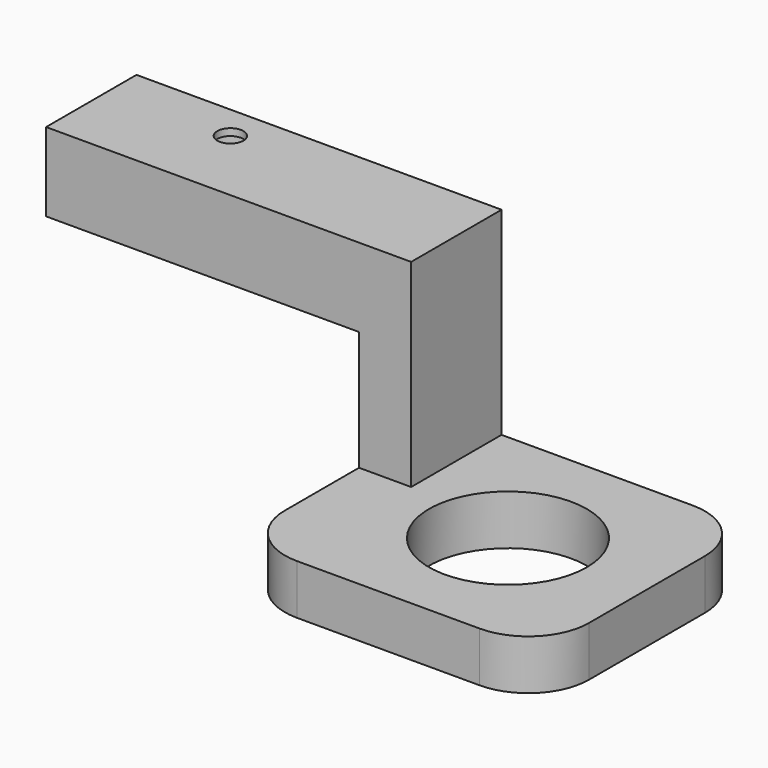
from build123d import *

# Parameters (mm, degrees)
F0_W     = 6
F0_H     = 13
F0_W_2   = 36
F0_R     = 3
F0_R_2   = 1.5
F1_DEPTH = 0.8
F2_DEPTH = 22
F3_DEPTH = 8.25
F4_R     = 13
F4_W     = 6
F4_H     = 13
F4_R_2   = 9.08
F5_DEPTH = 5.75
F6_R     = 7


# Not quite as in the source:
# - a feature names something its author has since deleted; it is built from what else it names


with BuildPart() as f1:
    # F0 (on Top) → F1 (new body)
    with BuildSketch(Plane.XY):
        with Locations((-3, 6.5)):
            Rectangle(F0_W, F0_H)
        with Locations((-24, 6.5)):
            Rectangle(F0_W_2, F0_H)
        with Locations((-28, 9)):
            Circle(F0_R, mode=Mode.SUBTRACT)
        with Locations((-28, 9)):
            Circle(F0_R)
        with Locations((-28, 9)):
            Circle(F0_R_2, mode=Mode.SUBTRACT)
    extrude(amount=F1_DEPTH)

    # F0 (on Top) → F2 (join)
    with BuildSketch(Plane.XY):
        with Locations((-3, 6.5)):
            Rectangle(F0_W, F0_H)
    extrude(amount=-F2_DEPTH)

    # F0 (on Top) → F3 (join)
    with BuildSketch(Plane.XY):
        with Locations((-24, 6.5)):
            Rectangle(F0_W_2, F0_H)
        with Locations((-28, 9)):
            Circle(F0_R, mode=Mode.SUBTRACT)
    extrude(amount=-F3_DEPTH)

    # F4 (on face) → F5 (join)
    with BuildSketch(Plane(origin=(0, 0, -22), x_dir=(1, 0, 0), z_dir=(0, 0, -1))):
        Polygon((29, 17.66), (-6, 17.66), (-6, 0), (0, 0), (0, -13), (17.6005885005, -13), (29, -13), align=None)
        with Locations((13, 2.33)):
            Circle(F4_R, mode=Mode.SUBTRACT)
        with Locations((-3, -6.5)):
            Rectangle(F4_W, F4_H)
        with Locations((13, 2.33)):
            Circle(F4_R)
        with Locations((13, 2.33)):
            Circle(F4_R_2, mode=Mode.SUBTRACT)
    extrude(amount=F5_DEPTH)

    # F6
    f6_edges = [f1.edges().sort_by_distance(p)[0] for p in [
        (-6, -17.66, -24.875),
        (29, -17.66, -24.875),
        (29, 13, -24.875),
    ]]
    fillet(f6_edges, radius=F6_R)


solid = f1.part
